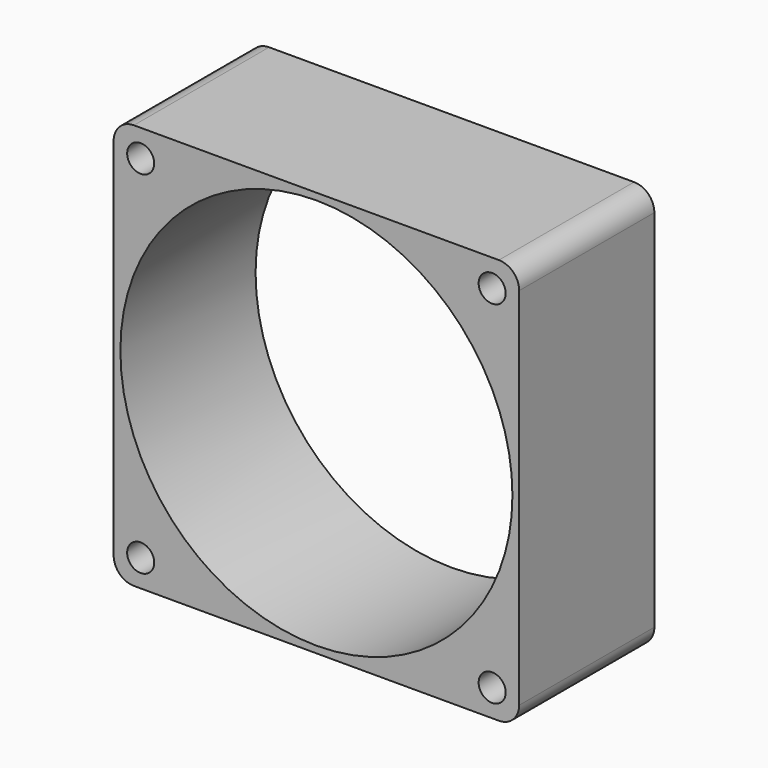
from build123d import *

# Parameters (mm, degrees)
F0_R     = 2
F0_R_2   = 29
F1_DEPTH = 25


# Not quite as in the source:
# - a feature of the source that left no trace in its solid (it failed there, or was rolled back) is left out


with BuildPart() as f1:
    # F0 (on Front) → F1 (new body)
    with BuildSketch(Plane.XZ):
        with BuildLine():
            ThreePointArc((0, 3), (0.8786796564, 0.8786796564), (3, 0))
            Line((3, 0), (57, 0))
            ThreePointArc((57, 0), (59.1213203436, 0.8786796564), (60, 3))
            Line((60, 3), (60, 57))
            ThreePointArc((60, 57), (59.1213203436, 59.1213203436), (57, 60))
            Line((57, 60), (3, 60))
            ThreePointArc((3, 60), (0.8786796564, 59.1213203436), (0, 57))
            Line((0, 57), (0, 3))
        make_face()
        with Locations((4, 4)):
            Circle(F0_R, mode=Mode.SUBTRACT)
        with Locations((56, 4)):
            Circle(F0_R, mode=Mode.SUBTRACT)
        with Locations((4, 56)):
            Circle(F0_R, mode=Mode.SUBTRACT)
        with Locations((30, 30)):
            Circle(F0_R_2, mode=Mode.SUBTRACT)
        with Locations((56, 56)):
            Circle(F0_R, mode=Mode.SUBTRACT)
    extrude(amount=F1_DEPTH)


solid = f1.part
